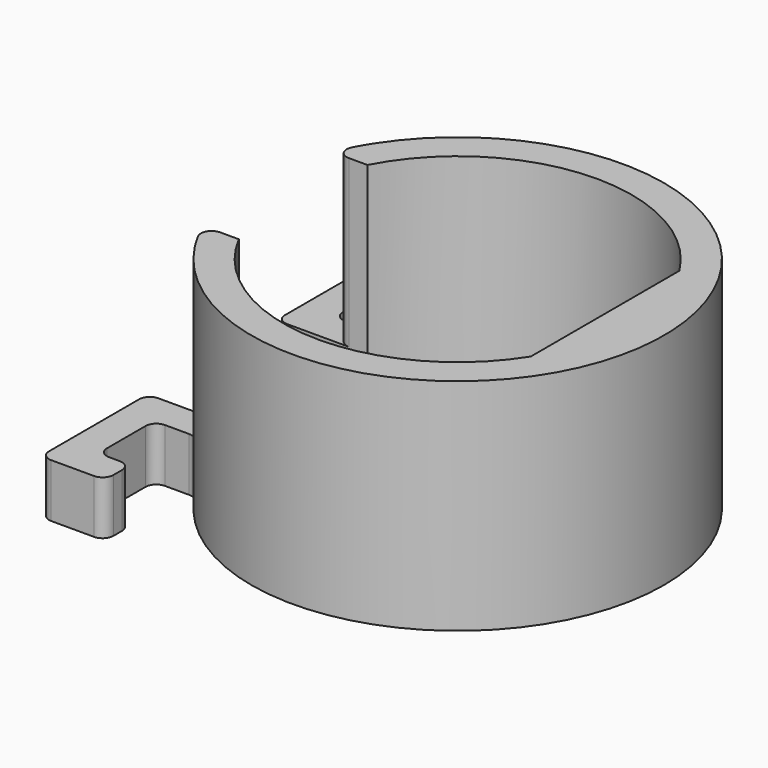
from build123d import *

# Parameters (mm, degrees)
F1_DEPTH    = 8.2
F2_DEPTH    = 1.2
F3_DEPTH    = 2
F4_R        = 0.4
F5_T1_DEPTH = 2
F5_T3_DEPTH = 4


# Not quite as in the source:
# - a fillet or chamfer that OpenCascade refuses, or shapes differently, is made with other operations: its cross-section is extruded or revolved along the edge and cut away or added
# - a feature names something its author has since deleted; it is built from what else it names


with BuildPart() as f1:
    # F0 (on Top) → F1 (new body)
    with BuildSketch(Plane.XY):
        with BuildLine():
            Line((-5.7662812973, -3), (-7.0915442606, -3))
            ThreePointArc((-7.0915442606, -3), (-6.7991383758, -3.6140997975), (-6.4536811201, -4.2))
            ThreePointArc((-6.4536811201, -4.2), (7.7, 0), (-6.4536811201, 4.2))
            ThreePointArc((-6.4536811201, 4.2), (-6.7991383758, 3.6140997975), (-7.0915442606, 3))
            Line((-7.0915442606, 3), (-5.7662812973, 3))
            ThreePointArc((-5.7662812973, 3), (-0.2675331935, 6.4944919732), (5.5, 3.4641016151))
            ThreePointArc((5.5, 3.4641016151), (6.5, 0), (5.5, -3.4641016151))
            ThreePointArc((5.5, -3.4641016151), (-0.2675331935, -6.4944919732), (-5.7662812973, -3))
        make_face()
        with BuildLine():
            Line((5.5, 3.4641016151), (5.5, -3.4641016151))
            ThreePointArc((5.5, -3.4641016151), (6.5, 0), (5.5, 3.4641016151))
        make_face()
    extrude(amount=F1_DEPTH)

    # F0 (on Top) → F2 (join)
    with BuildSketch(Plane.XY):
        with BuildLine():
            Line((0, -3), (-5.7662812973, -3))
            ThreePointArc((-5.7662812973, -3), (-0.2675331935, -6.4944919732), (5.5, -3.4641016151))
            Line((5.5, -3.4641016151), (5.5, 3.4641016151))
            ThreePointArc((5.5, 3.4641016151), (-0.2675331935, 6.4944919732), (-5.7662812973, 3))
            Line((-5.7662812973, 3), (0, 3))
            ThreePointArc((0, 3), (3, 0), (0, -3))
        make_face()
        with BuildLine():
            Line((5.5, 3.4641016151), (5.5, -3.4641016151))
            ThreePointArc((5.5, -3.4641016151), (6.5, 0), (5.5, 3.4641016151))
        make_face()
    extrude(amount=F2_DEPTH)

    # F0 (on Top) → F3 (join)
    with BuildSketch(Plane.XY):
        with BuildLine():
            ThreePointArc((-7.0915442606, 3), (-6.7991383758, 3.6140997975), (-6.4536811201, 4.2))
            Line((-6.4536811201, 4.2), (-7.9657880694, 4.2))
            Line((-7.9657880694, 4.2), (-7.9657880694, 6.8))
            Line((-7.9657880694, 6.8), (-6.7657880694, 6.8))
            Line((-6.7657880694, 6.8), (-6.7657880694, 8))
            Line((-6.7657880694, 8), (-7.9657880694, 8))
            Line((-7.9657880694, 8), (-9.1657880694, 8))
            Line((-9.1657880694, 8), (-9.1657880694, 3))
            Line((-9.1657880694, 3), (-7.0915442606, 3))
        make_face()
        with BuildLine():
            ThreePointArc((-6.4536811201, -4.2), (-6.7991383758, -3.6140997975), (-7.0915442606, -3))
            Line((-7.0915442606, -3), (-9.1657880694, -3))
            Line((-9.1657880694, -3), (-9.1657880694, -8))
            Line((-9.1657880694, -8), (-7.9657880694, -8))
            Line((-7.9657880694, -8), (-6.7657880694, -8))
            Line((-6.7657880694, -8), (-6.7657880694, -6.8))
            Line((-6.7657880694, -6.8), (-7.9657880694, -6.8))
            Line((-7.9657880694, -6.8), (-7.9657880694, -4.2))
            Line((-7.9657880694, -4.2), (-6.4536811201, -4.2))
        make_face()
    extrude(amount=F3_DEPTH)

    # F4
    f4_edges = [f1.edges().sort_by_distance(p)[0] for p in [
        (-7.091544, 3, 5.1),
        (-7.091544, -3, 5.1),
    ]]
    fillet(f4_edges, radius=F4_R)

    # F5: fillet of radius 0.4 on 14 edges, made by hand

    # F5_s2 → F5_t1 (join)
    with BuildSketch(Plane.XY):
        with BuildLine():
            ThreePointArc((-7.5657880694, 4.2), (-7.8486307818, 4.3171572875), (-7.9657880694, 4.6))
            Line((-7.9657880694, 4.6), (-7.9657880694, 4.2))
            Line((-7.9657880694, 4.2), (-7.5657880694, 4.2))
        make_face()
        with BuildLine():
            ThreePointArc((-6.3378446378, 4.3728395062), (-6.48115887, 4.2458360567), (-6.6670833203, 4.2))
            Line((-6.6670833203, 4.2), (-6.4536811201, 4.2))
            ThreePointArc((-6.4536811201, 4.2), (-6.3963467056, 4.2868110318), (-6.3378446378, 4.3728395062))
        make_face()
        with BuildLine():
            ThreePointArc((-6.3378446378, -4.3728395062), (-6.48115887, -4.2458360567), (-6.6670833203, -4.2))
            Line((-6.6670833203, -4.2), (-6.4536811201, -4.2))
            ThreePointArc((-6.4536811201, -4.2), (-6.3963467056, -4.2868110318), (-6.3378446378, -4.3728395062))
        make_face()
        with BuildLine():
            ThreePointArc((-7.5657880694, -4.2), (-7.8486307818, -4.3171572875), (-7.9657880694, -4.6))
            Line((-7.9657880694, -4.6), (-7.9657880694, -4.2))
            Line((-7.9657880694, -4.2), (-7.5657880694, -4.2))
        make_face()
        with BuildLine():
            ThreePointArc((-7.9657880694, -6.4), (-7.8486307818, -6.6828427125), (-7.5657880694, -6.8))
            Line((-7.5657880694, -6.8), (-7.9657880694, -6.8))
            Line((-7.9657880694, -6.8), (-7.9657880694, -6.4))
        make_face()
        with BuildLine():
            ThreePointArc((-7.9657880694, 6.4), (-7.8486307818, 6.6828427125), (-7.5657880694, 6.8))
            Line((-7.5657880694, 6.8), (-7.9657880694, 6.8))
            Line((-7.9657880694, 6.8), (-7.9657880694, 6.4))
        make_face()
    extrude(amount=F5_T1_DEPTH)

    # F5_s4 → F5_t3 (cut)
    with BuildSketch(Plane.XY.offset(-1)):
        with BuildLine():
            ThreePointArc((-8.7657880694, -8), (-9.0486307818, -7.8828427125), (-9.1657880694, -7.6))
            Line((-9.1657880694, -7.6), (-9.1657880694, -8))
            Line((-9.1657880694, -8), (-8.7657880694, -8))
        make_face()
        with BuildLine():
            ThreePointArc((-8.7657880694, -3), (-9.0486307818, -3.1171572875), (-9.1657880694, -3.4))
            Line((-9.1657880694, -3.4), (-9.1657880694, -3))
            Line((-9.1657880694, -3), (-8.7657880694, -3))
        make_face()
        with BuildLine():
            ThreePointArc((-8.7657880694, 3), (-9.0486307818, 3.1171572875), (-9.1657880694, 3.4))
            Line((-9.1657880694, 3.4), (-9.1657880694, 3))
            Line((-9.1657880694, 3), (-8.7657880694, 3))
        make_face()
        with BuildLine():
            ThreePointArc((-8.7657880694, 8), (-9.0486307818, 7.8828427125), (-9.1657880694, 7.6))
            Line((-9.1657880694, 7.6), (-9.1657880694, 8))
            Line((-9.1657880694, 8), (-8.7657880694, 8))
        make_face()
        with BuildLine():
            ThreePointArc((-7.1657880694, 6.8), (-6.8829453569, 6.9171572875), (-6.7657880694, 7.2))
            Line((-6.7657880694, 7.2), (-6.7657880694, 6.8))
            Line((-6.7657880694, 6.8), (-7.1657880694, 6.8))
        make_face()
        with BuildLine():
            ThreePointArc((-6.7657880694, -7.6), (-6.8829453569, -7.8828427125), (-7.1657880694, -8))
            Line((-7.1657880694, -8), (-6.7657880694, -8))
            Line((-6.7657880694, -8), (-6.7657880694, -7.6))
        make_face()
        with BuildLine():
            ThreePointArc((-7.1657880694, -6.8), (-6.8829453569, -6.9171572875), (-6.7657880694, -7.2))
            Line((-6.7657880694, -7.2), (-6.7657880694, -6.8))
            Line((-6.7657880694, -6.8), (-7.1657880694, -6.8))
        make_face()
        with BuildLine():
            ThreePointArc((-6.7657880694, 7.6), (-6.8829453569, 7.8828427125), (-7.1657880694, 8))
            Line((-7.1657880694, 8), (-6.7657880694, 8))
            Line((-6.7657880694, 8), (-6.7657880694, 7.6))
        make_face()
    extrude(amount=F5_T3_DEPTH, mode=Mode.SUBTRACT)


solid = f1.part
